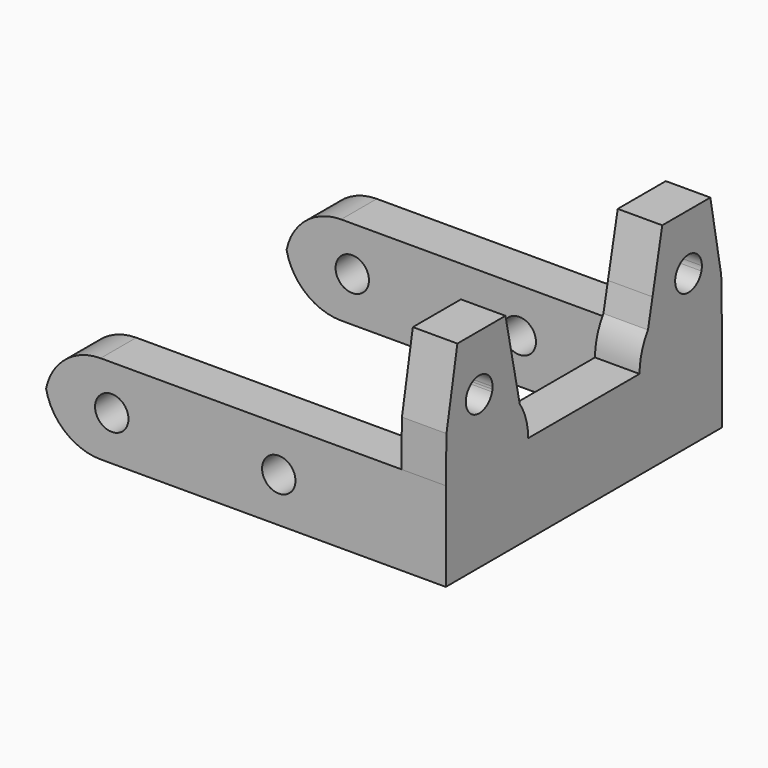
from build123d import *

# Parameters (mm, degrees)
F0_W        = 32
F0_H        = 4
F1_DEPTH    = 8
F3_DEPTH    = 4
F4_DEPTH    = 25
F5_R        = 1.5
F6_DEPTH    = 40
F7_T1_DEPTH = 29
F7_T3_DEPTH = 29


# Not quite as in the source:
# - a fillet or chamfer that OpenCascade refuses, or shapes differently, is made with other operations: its cross-section is extruded or revolved along the edge and cut away or added


with BuildPart() as f1:
    # F0 (on Top) → F1 (new body)
    with BuildSketch(Plane.XY):
        with Locations((-2, 13.5)):
            Rectangle(F0_W, F0_H)
        Polygon((14, 11.5), (14, -11.5), (14, -15.5), (18, -15.5), (18, 0), (18, 15.5), (14, 15.5), align=None)
        with Locations((-2, -13.5)):
            Rectangle(F0_W, F0_H)
    extrude(amount=F1_DEPTH)

    # F2 (on face) → F3 (join, through all)
    with BuildSketch(Plane.YZ.offset(18)):
        with BuildLine():
            Line((-15.4216540828, 12.0949916113), (-15.5, 8))
            Line((-15.5, 8), (-6.25, 8))
            ThreePointArc((-6.25, 8), (-6.4923756022, 9.6147401314), (-7.1981402517, 11.0871625858))
            ThreePointArc((-7.1981402517, 11.0871625858), (-8.5517740167, 12.4745223834), (-10.3026318448, 13.3061403509))
            ThreePointArc((-10.3026318448, 13.3061403509), (-11.75, 12.2), (-13.1973681552, 13.3061403509))
            ThreePointArc((-13.1973681552, 13.3061403509), (-14.3801744212, 12.8303397928), (-15.4216540828, 12.0949916113))
        make_face()
        with BuildLine():
            Line((6.25, 8), (11.75, 8))
            Line((11.75, 8), (15.5, 8))
            Line((15.5, 8), (15.4216540828, 12.0949916113))
            ThreePointArc((15.4216540828, 12.0949916113), (14.3801744212, 12.8303397928), (13.1973681552, 13.3061403509))
            ThreePointArc((13.1973681552, 13.3061403509), (11.75, 12.2), (10.3026318448, 13.3061403509))
            ThreePointArc((10.3026318448, 13.3061403509), (8.5517740167, 12.4745223834), (7.1981402517, 11.0871625858))
            ThreePointArc((7.1981402517, 11.0871625858), (6.4923756022, 9.6147401314), (6.25, 8))
        make_face()
        with BuildLine():
            Line((-14.1999293119, 18.7123082578), (-15.4216540828, 12.0949916113))
            ThreePointArc((-15.4216540828, 12.0949916113), (-14.3801744212, 12.8303397928), (-13.1973681552, 13.3061403509))
            ThreePointArc((-13.1973681552, 13.3061403509), (-11.9486803553, 15.1867838163), (-10.25, 13.7))
            ThreePointArc((-10.25, 13.7), (-10.2533520267, 13.5997760311), (-10.2633931253, 13.5))
            Line((-10.2633931253, 13.5), (-7.7054746686, 13.5))
            Line((-7.7054746686, 13.5), (-8.8014388457, 18.7123082578))
            Line((-8.8014388457, 18.7123082578), (-14.1999293119, 18.7123082578))
        make_face()
        with BuildLine():
            ThreePointArc((-10.3026318448, 13.3061403509), (-8.5517740167, 12.4745223834), (-7.1981402517, 11.0871625858))
            Line((-7.1981402517, 11.0871625858), (-7.7054746686, 13.5))
            Line((-7.7054746686, 13.5), (-10.2633931253, 13.5))
            ThreePointArc((-10.2633931253, 13.5), (-10.2798136989, 13.4024227159), (-10.3026318448, 13.3061403509))
        make_face()
        with BuildLine():
            ThreePointArc((13.1973681552, 13.3061403509), (14.3801744212, 12.8303397928), (15.4216540828, 12.0949916113))
            Line((15.4216540828, 12.0949916113), (14.1999293119, 18.7123082578))
            Line((14.1999293119, 18.7123082578), (8.8014388457, 18.7123082578))
            Line((8.8014388457, 18.7123082578), (7.7054746686, 13.5))
            Line((7.7054746686, 13.5), (10.2633931253, 13.5))
            ThreePointArc((10.2633931253, 13.5), (11.6497760311, 15.1966479733), (13.25, 13.7))
            ThreePointArc((13.25, 13.7), (13.2367838163, 13.5013196447), (13.1973681552, 13.3061403509))
        make_face()
        with BuildLine():
            Line((7.7054746686, 13.5), (7.1981402517, 11.0871625858))
            ThreePointArc((7.1981402517, 11.0871625858), (8.5517740167, 12.4745223834), (10.3026318448, 13.3061403509))
            ThreePointArc((10.3026318448, 13.3061403509), (10.2798136989, 13.4024227159), (10.2633931253, 13.5))
            Line((10.2633931253, 13.5), (7.7054746686, 13.5))
        make_face()
    extrude(amount=-F3_DEPTH)

    # F2 (on face) → F4 (cut)
    with BuildSketch(Plane.YZ.offset(18)):
        with BuildLine():
            ThreePointArc((10.2633931253, 13.5), (10.2798136989, 13.4024227159), (10.3026318448, 13.3061403509))
            ThreePointArc((10.3026318448, 13.3061403509), (11.0198534153, 13.4513196535), (11.75, 13.5))
            Line((11.75, 13.5), (10.2633931253, 13.5))
        make_face()
        with BuildLine():
            ThreePointArc((11.75, 13.5), (11.0198534153, 13.4513196535), (10.3026318448, 13.3061403509))
            ThreePointArc((10.3026318448, 13.3061403509), (11.75, 12.2), (13.1973681552, 13.3061403509))
            ThreePointArc((13.1973681552, 13.3061403509), (12.4801465847, 13.4513196535), (11.75, 13.5))
        make_face()
        with BuildLine():
            ThreePointArc((11.75, 13.5), (12.4801465847, 13.4513196535), (13.1973681552, 13.3061403509))
            ThreePointArc((13.1973681552, 13.3061403509), (13.2367838163, 13.5013196447), (13.25, 13.7))
            ThreePointArc((13.25, 13.7), (11.6497760311, 15.1966479733), (10.2633931253, 13.5))
            Line((10.2633931253, 13.5), (11.75, 13.5))
        make_face()
        with BuildLine():
            ThreePointArc((-11.75, 13.5), (-12.4801465847, 13.4513196535), (-13.1973681552, 13.3061403509))
            ThreePointArc((-13.1973681552, 13.3061403509), (-11.75, 12.2), (-10.3026318448, 13.3061403509))
            ThreePointArc((-10.3026318448, 13.3061403509), (-11.0198534153, 13.4513196535), (-11.75, 13.5))
        make_face()
        with BuildLine():
            ThreePointArc((-11.75, 13.5), (-11.0198534153, 13.4513196535), (-10.3026318448, 13.3061403509))
            ThreePointArc((-10.3026318448, 13.3061403509), (-10.2798136989, 13.4024227159), (-10.2633931253, 13.5))
            Line((-10.2633931253, 13.5), (-11.75, 13.5))
        make_face()
        with BuildLine():
            ThreePointArc((-10.25, 13.7), (-11.9486803553, 15.1867838163), (-13.1973681552, 13.3061403509))
            ThreePointArc((-13.1973681552, 13.3061403509), (-12.4801465847, 13.4513196535), (-11.75, 13.5))
            Line((-11.75, 13.5), (-10.2633931253, 13.5))
            ThreePointArc((-10.2633931253, 13.5), (-10.2533520267, 13.5997760311), (-10.25, 13.7))
        make_face()
    extrude(amount=-F4_DEPTH, mode=Mode.SUBTRACT)

    # F5 (on face) → F6 (cut)
    with BuildSketch(Plane.XZ.offset(15.5)):
        with Locations((-12, 4)):
            Circle(F5_R)
        with Locations((3, 4)):
            Circle(F5_R)
    extrude(amount=-F6_DEPTH, mode=Mode.SUBTRACT)

    # F7: fillet of radius 5 on 4 edges, made by hand

    # F7_s2 → F7_t1 (cut)
    with BuildSketch(Plane.XZ.offset(-1)):
        with BuildLine():
            ThreePointArc((-18, 3), (-16.5355339059, 6.5355339059), (-13, 8))
            Line((-13, 8), (-18, 8))
            Line((-18, 8), (-18, 3))
        make_face()
        with BuildLine():
            ThreePointArc((-13, 0), (-16.5355339059, 1.4644660941), (-18, 5))
            Line((-18, 5), (-18, 0))
            Line((-18, 0), (-13, 0))
        make_face()
    extrude(amount=F7_T1_DEPTH, mode=Mode.SUBTRACT)

    # F7_s4 → F7_t3 (cut)
    with BuildSketch(Plane.XZ.offset(-28)):
        with BuildLine():
            ThreePointArc((-18, 3), (-16.5355339059, 6.5355339059), (-13, 8))
            Line((-13, 8), (-18, 8))
            Line((-18, 8), (-18, 3))
        make_face()
        with BuildLine():
            ThreePointArc((-18, 5), (-16.5355339059, 1.4644660941), (-13, 0))
            Line((-13, 0), (-18, 0))
            Line((-18, 0), (-18, 5))
        make_face()
    extrude(amount=F7_T3_DEPTH, mode=Mode.SUBTRACT)


solid = f1.part
